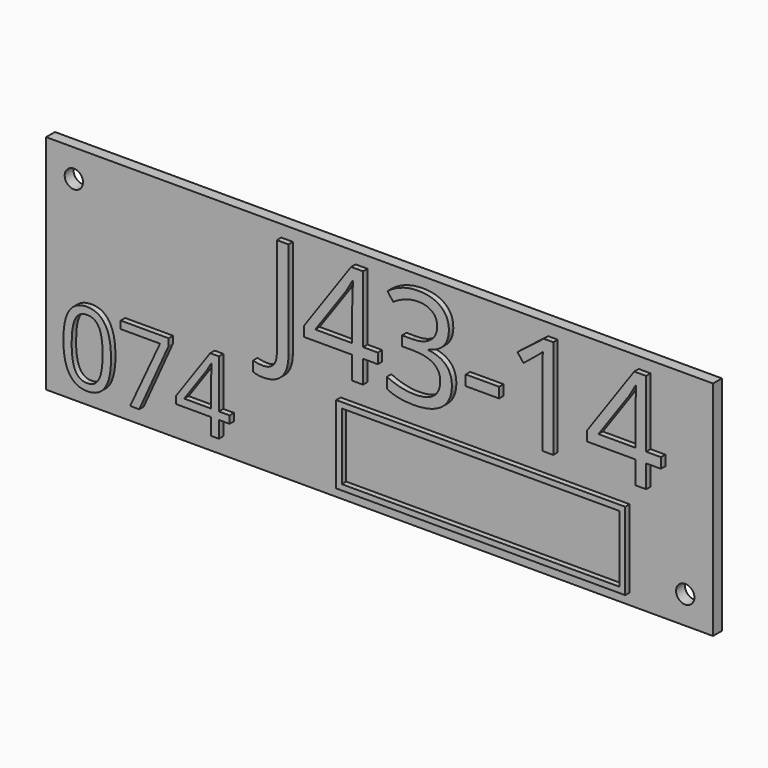
from build123d import *

# Parameters (mm, degrees)
F0_W         = 120
F0_H         = 40
F1_DEPTH     = 2
F3_D         = 3.3
F4_TEXT_SIZE = 25.0117242457
F5_DEPTH     = 1
F6_TEXT_SIZE = 18.1818181818
F7_DEPTH     = 1
F8_W         = 52
F8_H         = 14
F8_W_2       = 49.99999962
F8_H_2       = 11.99999962
F9_DEPTH     = 1


# Not quite as in the source:
# - Text() gives the source's letters only with a copy of the font that has no kerning and outlines rounded to 1/6400 em; it was checked with that copy


with BuildPart() as f1:
    # F0 (on Front) → F1 (new body)
    with BuildSketch(Plane.XZ):
        Rectangle(F0_W, F0_H)
    extrude(amount=F1_DEPTH)

    # F3 (through all)
    with Locations(Plane.XZ.offset(2)):
        with Locations((-55, 15), (55, -15)):
            Hole(F3_D / 2)

    # F4 (on face) → F5 (join)
    with BuildSketch(Plane.XZ.offset(2)):
        with Locations((-20, 0)):
            Text('J43-14', F4_TEXT_SIZE, font='Open Sans', text_align=(TextAlign.LEFT, TextAlign.BOTTOM))
    extrude(amount=F5_DEPTH)

    # F6 (on face) → F7 (join)
    with BuildSketch(Plane.XZ.offset(2)):
        with Locations((-57, -17)):
            Text('074', F6_TEXT_SIZE, font='Open Sans', text_align=(TextAlign.LEFT, TextAlign.BOTTOM))
    extrude(amount=F7_DEPTH)

    # F8 (on face) → F9 (join)
    with BuildSketch(Plane.XZ.offset(2)):
        with Locations((19, -11)):
            Rectangle(F8_W, F8_H)
        with Locations((19, -11)):
            Rectangle(F8_W_2, F8_H_2, mode=Mode.SUBTRACT)
    extrude(amount=F9_DEPTH)


solid = f1.part
